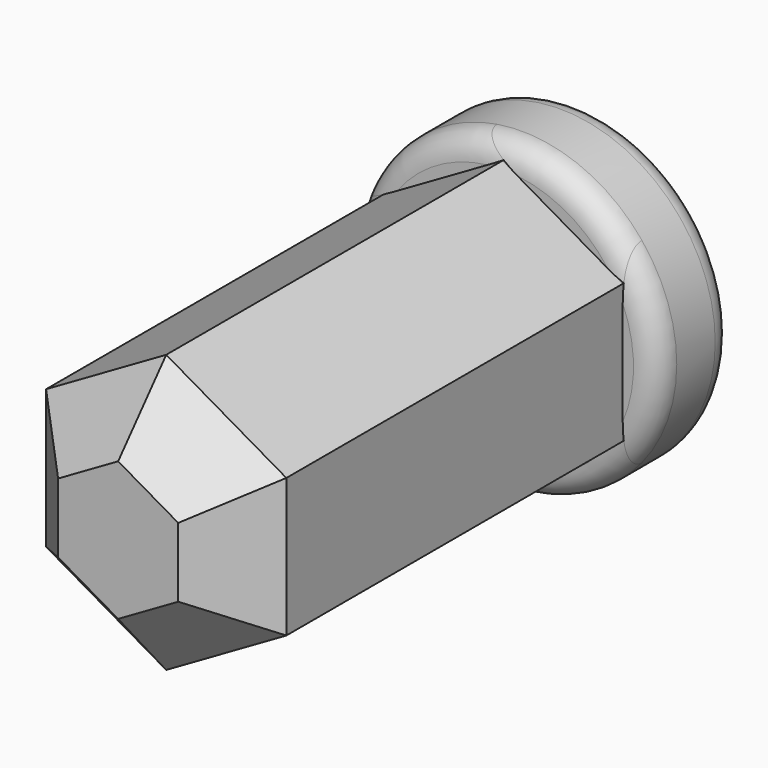
from build123d import *

# Parameters (mm, degrees)
F1_DEPTH = 50.8
F2_R     = 16.3806904911
F3_DEPTH = 10.16
F6_SIZE  = 6.35


# Not quite as in the source:
# - a fillet or chamfer that OpenCascade refuses, or shapes differently, is made with other operations: its cross-section is extruded or revolved along the edge and cut away or added


with BuildPart() as f1:
    # F0 (on Front) → F1 (new body)
    with BuildSketch(Plane.XZ):
        Polygon((12.7, -7.3323484187), (12.7, 7.3323484187), (0, 14.6646968374), (-12.7, 7.3323484187), (-12.7, -7.3323484187), (0, -14.6646968374), align=None)
    extrude(amount=F1_DEPTH)

    # F2 (on Front) + F1_face (on face) + F1_face1 (on face) → F3 (join)
    with BuildSketch(Plane.XZ):
        Circle(F2_R)
    with BuildSketch(Plane(origin=(0, 0, 0), x_dir=(1, 0, 0), z_dir=(0, 1, 0))):
        Polygon((12.7, -7.3323484187), (12.7, 7.3323484187), (0, 14.6646968374), (-12.7, 7.3323484187), (-12.7, -7.3323484187), (0, -14.6646968374), align=None)
    with BuildSketch(Plane.XZ.offset(50.8)):
        Polygon((12.7, -7.3323484187), (12.7, 7.3323484187), (0, 14.6646968374), (-12.7, 7.3323484187), (-12.7, -7.3323484187), (0, -14.6646968374), align=None)
    extrude(amount=-F3_DEPTH, dir=(0, -1, 0))

    # F4: fillet of radius 2.54 on 3 edges, made by hand

    # F4_s1 → F4_t2 (revolve, cut)
    with BuildSketch(Plane.XY):
        with BuildLine():
            ThreePointArc((16.3806904911, 7.62), (15.6367417153, 9.4160512242), (13.8406904911, 10.16))
            Line((13.8406904911, 10.16), (16.3806904911, 10.16))
            Line((16.3806904911, 10.16), (16.3806904911, 7.62))
        make_face()
    revolve(axis=Axis((0, 10.16, 0), (0, -1, 0)), mode=Mode.SUBTRACT)


with BuildPart() as f4_tool4:
    # F4_s5 → F4_t6 (revolve)
    with BuildSketch(Plane.XY):
        with BuildLine():
            ThreePointArc((13.8406904911, 0), (15.6367417153, 0.7439487758), (16.3806904911, 2.54))
            Line((16.3806904911, 2.54), (16.3806904911, 0))
            Line((16.3806904911, 0), (13.8406904911, 0))
        make_face()
    revolve(axis=Axis((0, 0, 0), (0, -1, 0)))

    split(bisect_by=Plane.YZ.offset(12.7), keep=Keep.TOP)


with BuildPart() as f1_1:
    add(f1.part)

    # F4_t3: cut F4_tool4
    add(f4_tool4.part, mode=Mode.SUBTRACT)


with BuildPart() as f4_tool9:
    # F4_s10 → F4_t11 (revolve)
    with BuildSketch(Plane.XY):
        with BuildLine():
            ThreePointArc((13.8406904911, 0), (15.6367417153, 0.7439487758), (16.3806904911, 2.54))
            Line((16.3806904911, 2.54), (16.3806904911, 0))
            Line((16.3806904911, 0), (13.8406904911, 0))
        make_face()
    revolve(axis=Axis((0, 0, 0), (0, -1, 0)))

    split(bisect_by=Plane(origin=(6.35, 0, 10.9985226281), x_dir=(0, 1, 0), z_dir=(0.5, 0, 0.8660254038)), keep=Keep.TOP)


with BuildPart() as f1_2:
    add(f1_1.part)

    # F4_t8: cut F4_tool9
    add(f4_tool9.part, mode=Mode.SUBTRACT)


with BuildPart() as f4_tool14:
    # F4_s15 → F4_t16 (revolve)
    with BuildSketch(Plane.XY):
        with BuildLine():
            ThreePointArc((13.8406904911, 0), (15.6367417153, 0.7439487758), (16.3806904911, 2.54))
            Line((16.3806904911, 2.54), (16.3806904911, 0))
            Line((16.3806904911, 0), (13.8406904911, 0))
        make_face()
    revolve(axis=Axis((0, 0, 0), (0, -1, 0)))

    split(bisect_by=Plane(origin=(6.35, 0, -10.9985226281), x_dir=(0, 1, 0), z_dir=(0.5, 0, -0.8660254038)), keep=Keep.TOP)


with BuildPart() as f1_3:
    add(f1_2.part)

    # F4_t13: cut F4_tool14
    add(f4_tool14.part, mode=Mode.SUBTRACT)


with BuildPart() as f4_tool19:
    # F4_s20 → F4_t21 (revolve)
    with BuildSketch(Plane.XY):
        with BuildLine():
            ThreePointArc((13.8406904911, 0), (15.6367417153, 0.7439487758), (16.3806904911, 2.54))
            Line((16.3806904911, 2.54), (16.3806904911, 0))
            Line((16.3806904911, 0), (13.8406904911, 0))
        make_face()
    revolve(axis=Axis((0, 0, 0), (0, -1, 0)))

    split(bisect_by=Plane(origin=(-6.35, 0, 10.9985226281), x_dir=(0, 1, 0), z_dir=(-0.5, 0, 0.8660254038)), keep=Keep.TOP)


with BuildPart() as f1_4:
    add(f1_3.part)

    # F4_t18: cut F4_tool19
    add(f4_tool19.part, mode=Mode.SUBTRACT)


with BuildPart() as f4_tool24:
    # F4_s25 → F4_t26 (revolve)
    with BuildSketch(Plane.XY):
        with BuildLine():
            ThreePointArc((13.8406904911, 0), (15.6367417153, 0.7439487758), (16.3806904911, 2.54))
            Line((16.3806904911, 2.54), (16.3806904911, 0))
            Line((16.3806904911, 0), (13.8406904911, 0))
        make_face()
    revolve(axis=Axis((0, 0, 0), (0, -1, 0)))

    split(bisect_by=Plane(origin=(-6.35, 0, -10.9985226281), x_dir=(0, 1, 0), z_dir=(-0.5, 0, -0.8660254038)), keep=Keep.TOP)


with BuildPart() as f1_5:
    add(f1_4.part)

    # F4_t23: cut F4_tool24
    add(f4_tool24.part, mode=Mode.SUBTRACT)


with BuildPart() as f4_tool29:
    # F4_s30 → F4_t31 (revolve)
    with BuildSketch(Plane.XY):
        with BuildLine():
            ThreePointArc((13.8406904911, 0), (15.6367417153, 0.7439487758), (16.3806904911, 2.54))
            Line((16.3806904911, 2.54), (16.3806904911, 0))
            Line((16.3806904911, 0), (13.8406904911, 0))
        make_face()
    revolve(axis=Axis((0, 0, 0), (0, -1, 0)))

    split(bisect_by=Plane.YZ.offset(-12.7), keep=Keep.BOTTOM)


with BuildPart() as f1_6:
    add(f1_5.part)

    # F4_t28: cut F4_tool29
    add(f4_tool29.part, mode=Mode.SUBTRACT)

    # F6
    f6_edges = [f1_6.edges().sort_by_distance(p)[0] for p in [
        (12.7, -50.8, 0),
        (6.35, -50.8, 10.998523),
        (-6.35, -50.8, 10.998523),
        (-12.7, -50.8, 0),
        (-6.35, -50.8, -10.998523),
        (6.35, -50.8, -10.998523),
    ]]
    chamfer(f6_edges, length=F6_SIZE)


solid = f1_6.part
